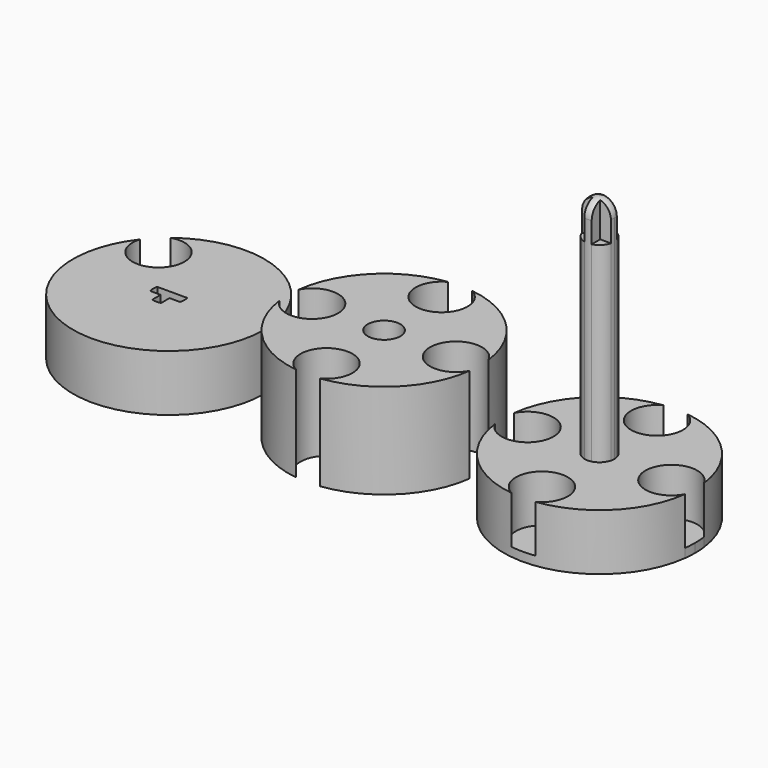
from build123d import *

# Parameters (mm, degrees)
F3_R             = 5.5
F6_DEPTH         = 32
F7_DEPTH         = 32.001
F7_COPIES_COUNT  = 4
F8_DEPTH         = 19
F9_DEPTH         = 95.5
F10_DEPTH        = 83.5
F11_T2_ANGLE     = 315.5011633423
F11_T4_ANGLE     = 315.5011633423
F11_T6_ANGLE     = 315.5011633423
F12_START        = 3
F12_DEPTH        = 92.5010001001
F12_COPIES_COUNT = 4
F13_START        = 3
F13_DEPTH        = 92.5010001001
F14_DEPTH        = 19
F15_DEPTH        = 6.2
F16_DEPTH        = 3


# Not quite as in the source:
# - a fillet or chamfer that OpenCascade refuses, or shapes differently, is made with other operations: its cross-section is extruded or revolved along the edge and cut away or added
# - a pattern or mirror of a feature is missing from the dataset's text; its kind, count and spacing are read off the source's solid
# - a feature names something its author has since deleted; it is built from what else it names


with BuildPart() as f6:
    # F3 (on Top) → F6 (new body)
    with BuildSketch(Plane.XY):
        with BuildLine():
            ThreePointArc((32.0321912081, -4), (15.5, 0), (32.0321912081, 4))
            ThreePointArc((32.0321912081, 4), (-32.2809738638, 0), (32.0321912081, -4))
        make_face()
        Circle(F3_R, mode=Mode.SUBTRACT)
        with BuildLine():
            ThreePointArc((32.2809738638, 0), (32.218718168, 2.0038645669), (32.0321912081, 4))
            ThreePointArc((32.0321912081, 4), (15.5, 0), (32.0321912081, -4))
            ThreePointArc((32.0321912081, -4), (32.218718168, -2.0038645669), (32.2809738638, 0))
        make_face()
    extrude(amount=F6_DEPTH)

    # F3 (on Top) → F7 (cut, through all)
    with BuildSketch(Plane.XY):
        with BuildLine():
            ThreePointArc((32.2809738638, 0), (32.218718168, 2.0038645669), (32.0321912081, 4))
            ThreePointArc((32.0321912081, 4), (15.5, 0), (32.0321912081, -4))
            ThreePointArc((32.0321912081, -4), (32.218718168, -2.0038645669), (32.2809738638, 0))
        make_face()
    f7 = extrude(amount=F7_DEPTH, mode=Mode.SUBTRACT)

    # F7_copies: F7 ×4 about axis
    f7_copies_axis = Axis((0, 0, 0), (0, 0, 1))
    for i in range(1, F7_COPIES_COUNT):
        add(f7.rotate(f7_copies_axis, i * 360 / F7_COPIES_COUNT), mode=Mode.SUBTRACT)

    # F3 (on Top) → F13 (cut)
    with BuildSketch(Plane.XY.offset(F13_START)):
        with BuildLine():
            ThreePointArc((104.6643824017, -4), (104.8509093616, -2.0038645669), (104.9131650573, 0))
            ThreePointArc((104.9131650573, 0), (104.8509093616, 2.0038645669), (104.6643824017, 4))
            ThreePointArc((104.6643824017, 4), (88.1321911935, 0), (104.6643824017, -4))
        make_face()
    extrude(amount=F13_DEPTH, mode=Mode.SUBTRACT)


with BuildPart() as f8:
    # F3 (on Top) → F8 (new body)
    with BuildSketch(Plane.XY):
        with BuildLine():
            ThreePointArc((104.6643824017, -4), (88.1321911935, 0), (104.6643824017, 4))
            ThreePointArc((104.6643824017, 4), (40.3512173297, 0), (104.6643824017, -4))
        make_face()
        with BuildLine():
            ThreePointArc((77.4734203763, 1.25), (77.5923396749, 0.6300214624), (77.6321911935, 0))
            ThreePointArc((77.6321911935, 0), (77.5923396749, -0.6300214624), (77.4734203763, -1.25))
            ThreePointArc((77.4734203763, -1.25), (76.1677250995, -3.5355339059), (73.8821911935, -4.8412291828))
            ThreePointArc((73.8821911935, -4.8412291828), (72.6321911935, -5), (71.3821911935, -4.8412291828))
            ThreePointArc((71.3821911935, -4.8412291828), (69.0966572876, -3.5355339059), (67.7909620108, -1.25))
            ThreePointArc((67.7909620108, -1.25), (67.6321911935, 0), (67.7909620108, 1.25))
            ThreePointArc((67.7909620108, 1.25), (72.6321911935, 5), (77.4734203763, 1.25))
        make_face(mode=Mode.SUBTRACT)
        with BuildLine():
            ThreePointArc((73.8821911935, -4.8412291828), (76.1677250995, -3.5355339059), (77.4734203763, -1.25))
            Line((77.4734203763, -1.25), (73.8821911935, -1.25))
            Line((73.8821911935, -1.25), (73.8821911935, -4.8412291828))
        make_face()
        with BuildLine():
            Line((71.3821911935, -1.25), (67.7909620108, -1.25))
            ThreePointArc((67.7909620108, -1.25), (69.0966572876, -3.5355339059), (71.3821911935, -4.8412291828))
            Line((71.3821911935, -4.8412291828), (71.3821911935, -1.25))
        make_face()
        with BuildLine():
            ThreePointArc((104.6643824017, -4), (104.8509093616, -2.0038645669), (104.9131650573, 0))
            ThreePointArc((104.9131650573, 0), (104.8509093616, 2.0038645669), (104.6643824017, 4))
            ThreePointArc((104.6643824017, 4), (88.1321911935, 0), (104.6643824017, -4))
        make_face()
    extrude(amount=F8_DEPTH)

    # F3 (on Top) → F9 (join)
    with BuildSketch(Plane.XY):
        with BuildLine():
            ThreePointArc((77.4734203763, -1.25), (77.5923396749, -0.6300214624), (77.6321911935, 0))
            ThreePointArc((77.6321911935, 0), (77.5923396749, 0.6300214624), (77.4734203763, 1.25))
            Line((77.4734203763, 1.25), (67.7909620108, 1.25))
            ThreePointArc((67.7909620108, 1.25), (67.6321911935, 0), (67.7909620108, -1.25))
            Line((67.7909620108, -1.25), (71.3821911935, -1.25))
            Line((71.3821911935, -1.25), (71.3821911935, -4.8412291828))
            ThreePointArc((71.3821911935, -4.8412291828), (72.6321911935, -5), (73.8821911935, -4.8412291828))
            Line((73.8821911935, -4.8412291828), (73.8821911935, -1.25))
            Line((73.8821911935, -1.25), (77.4734203763, -1.25))
        make_face()
    extrude(amount=F9_DEPTH)

    # F3 (on Top) → F10 (join)
    with BuildSketch(Plane.XY):
        with BuildLine():
            Line((71.3821911935, -1.25), (67.7909620108, -1.25))
            ThreePointArc((67.7909620108, -1.25), (69.0966572876, -3.5355339059), (71.3821911935, -4.8412291828))
            Line((71.3821911935, -4.8412291828), (71.3821911935, -1.25))
        make_face()
        with BuildLine():
            ThreePointArc((73.8821911935, -4.8412291828), (76.1677250995, -3.5355339059), (77.4734203763, -1.25))
            Line((77.4734203763, -1.25), (73.8821911935, -1.25))
            Line((73.8821911935, -1.25), (73.8821911935, -4.8412291828))
        make_face()
        with BuildLine():
            Line((67.7909620108, 1.25), (77.4734203763, 1.25))
            ThreePointArc((77.4734203763, 1.25), (72.6321911935, 5), (67.7909620108, 1.25))
        make_face()
    extrude(amount=F10_DEPTH)

    # F11: fillet of radius 5 on 3 edges, made by hand

    # F11_s1 → F11_t2 (revolve, cut)
    with BuildSketch(Plane(origin=(62.2190839151, 25.4537619139, 0), x_dir=(0, 0, 1), z_dir=(0.925544348, 0.3786392212, 0))):
        with BuildLine():
            ThreePointArc((90.4990343146, 22.5009963057), (94.0351924681, 23.9655209949), (95.5003999068, 27.5013963057))
            Line((95.5003999068, 27.5013963057), (96.0005364913, 27.5013963057))
            Line((96.0005364913, 27.5013963057), (96.0001365685, 22.5013963057))
            Line((96.0001365685, 22.5013963057), (95.5, 22.0012597372))
            ThreePointArc((95.5, 22.0012597372), (92.9995171573, 22.0012597372), (90.4990343146, 22.0008597372))
            Line((90.4990343146, 22.0008597372), (90.4990343146, 22.5009963057))
        make_face()
    revolve(axis=Axis((72.6321911935, 0, 95.5), (0, 0, 1)), revolution_arc=F11_T2_ANGLE, mode=Mode.SUBTRACT)

    # F11_s3 → F11_t4 (revolve, cut)
    with BuildSketch(Plane(origin=(10.4131072784, -25.453761914, 0), x_dir=(0, 0, 1), z_dir=(0.3786392212, -0.925544348, 0))):
        with BuildLine():
            ThreePointArc((90.4990343146, -72.2247140449), (94.0351924681, -70.7601893557), (95.5003999068, -67.2243140449))
            Line((95.5003999068, -67.2243140449), (96.0005364913, -67.2243140449))
            Line((96.0005364913, -67.2243140449), (96.0001365685, -72.2243140449))
            Line((96.0001365685, -72.2243140449), (95.5, -72.7244506135))
            ThreePointArc((95.5, -72.7244506135), (92.9995171573, -72.7244506135), (90.4990343146, -72.7248506135))
            Line((90.4990343146, -72.7248506135), (90.4990343146, -72.2247140449))
        make_face()
    revolve(axis=Axis((72.6321911935, 0, 95.5), (0, 0, 1)), revolution_arc=F11_T4_ANGLE, mode=Mode.SUBTRACT)

    # F11_s5 → F11_t6 (revolve, cut)
    with BuildSketch(Plane(origin=(10.4131072784, 25.453761914, 0), x_dir=(0, 0, 1), z_dir=(-0.3786392212, -0.925544348, 0))):
        with BuildLine():
            ThreePointArc((90.4990343146, -62.2239140449), (94.0351924681, -63.6884387341), (95.5003999068, -67.2243140449))
            Line((95.5003999068, -67.2243140449), (96.0005364913, -67.2243140449))
            Line((96.0005364913, -67.2243140449), (96.0001365685, -62.2243140449))
            Line((96.0001365685, -62.2243140449), (95.5, -61.7241774764))
            ThreePointArc((95.5, -61.7241774764), (92.9995171573, -61.7241774764), (90.4990343146, -61.7237774764))
            Line((90.4990343146, -61.7237774764), (90.4990343146, -62.2239140449))
        make_face()
    revolve(axis=Axis((72.6321911935, 0, 95.5), (0, 0, -1)), revolution_arc=F11_T6_ANGLE, mode=Mode.SUBTRACT)

    # F3 (on Top) → F12 (cut)
    with BuildSketch(Plane.XY.offset(F12_START)):
        with BuildLine():
            ThreePointArc((104.6643824017, -4), (104.8509093616, -2.0038645669), (104.9131650573, 0))
            ThreePointArc((104.9131650573, 0), (104.8509093616, 2.0038645669), (104.6643824017, 4))
            ThreePointArc((104.6643824017, 4), (88.1321911935, 0), (104.6643824017, -4))
        make_face()
    f12 = extrude(amount=F12_DEPTH, mode=Mode.SUBTRACT)

    # F12_copies: F12 ×4 about axis
    f12_copies_axis = Axis((72.632191, 0, 0), (0, 0, 1))
    for i in range(1, F12_COPIES_COUNT):
        add(f12.rotate(f12_copies_axis, i * 360 / F12_COPIES_COUNT), mode=Mode.SUBTRACT)


with BuildPart() as f14:
    # F3 (on Top) → F14 (new body)
    with BuildSketch(Plane.XY):
        with BuildLine():
            ThreePointArc((-98.1107979378, 19.8217524948), (-83.1104313892, -30.5330600497), (-40.3512173297, 0))
            ThreePointArc((-40.3512173297, 0), (-58.4512920793, 28.9993685088), (-92.4539436883, 25.4786067443))
            ThreePointArc((-92.4539436883, 25.4786067443), (-83.5923463019, 10.9601551084), (-98.1107979378, 19.8217524948))
        make_face()
        with BuildLine():
            Line((-71.1321911935, 1.5), (-67.6010382442, 1.5))
            ThreePointArc((-67.6010382442, 1.5), (-67.3821911935, 0), (-67.6010382442, -1.5))
            Line((-67.6010382442, -1.5), (-71.1321911935, -1.5))
            Line((-71.1321911935, -1.5), (-71.1321911935, -5.0311529494))
            ThreePointArc((-71.1321911935, -5.0311529494), (-72.6321911935, -5.25), (-74.1321911935, -5.0311529494))
            Line((-74.1321911935, -5.0311529494), (-74.1321911935, -1.5))
            Line((-74.1321911935, -1.5), (-77.6633441429, -1.5))
            ThreePointArc((-77.6633441429, -1.5), (-77.8821911935, 0), (-77.6633441429, 1.5))
            Line((-77.6633441429, 1.5), (-74.1321911935, 1.5))
            Line((-74.1321911935, 1.5), (-71.1321911935, 1.5))
        make_face(mode=Mode.SUBTRACT)
    extrude(amount=F14_DEPTH)

    # F3 (on Top) → F15 (join)
    with BuildSketch(Plane.XY):
        with BuildLine():
            ThreePointArc((-67.6010382442, -1.5), (-67.3821911935, 0), (-67.6010382442, 1.5))
            Line((-67.6010382442, 1.5), (-71.1321911935, 1.5))
            Line((-71.1321911935, 1.5), (-74.1321911935, 1.5))
            Line((-74.1321911935, 1.5), (-77.6633441429, 1.5))
            ThreePointArc((-77.6633441429, 1.5), (-77.8821911935, 0), (-77.6633441429, -1.5))
            Line((-77.6633441429, -1.5), (-74.1321911935, -1.5))
            Line((-74.1321911935, -1.5), (-74.1321911935, -5.0311529494))
            ThreePointArc((-74.1321911935, -5.0311529494), (-72.6321911935, -5.25), (-71.1321911935, -5.0311529494))
            Line((-71.1321911935, -5.0311529494), (-71.1321911935, -1.5))
            Line((-71.1321911935, -1.5), (-67.6010382442, -1.5))
        make_face()
    extrude(amount=F15_DEPTH)

    # F3 (on Top) → F16 (join)
    with BuildSketch(Plane.XY):
        with BuildLine():
            ThreePointArc((-98.1107979378, 19.8217524948), (-83.5923463019, 10.9601551084), (-92.4539436883, 25.4786067443))
            ThreePointArc((-92.4539436883, 25.4786067443), (-95.4582867159, 22.8260955224), (-98.1107979378, 19.8217524948))
        make_face()
    extrude(amount=F16_DEPTH)


solid = Compound([f6.part, f8.part, f14.part])
